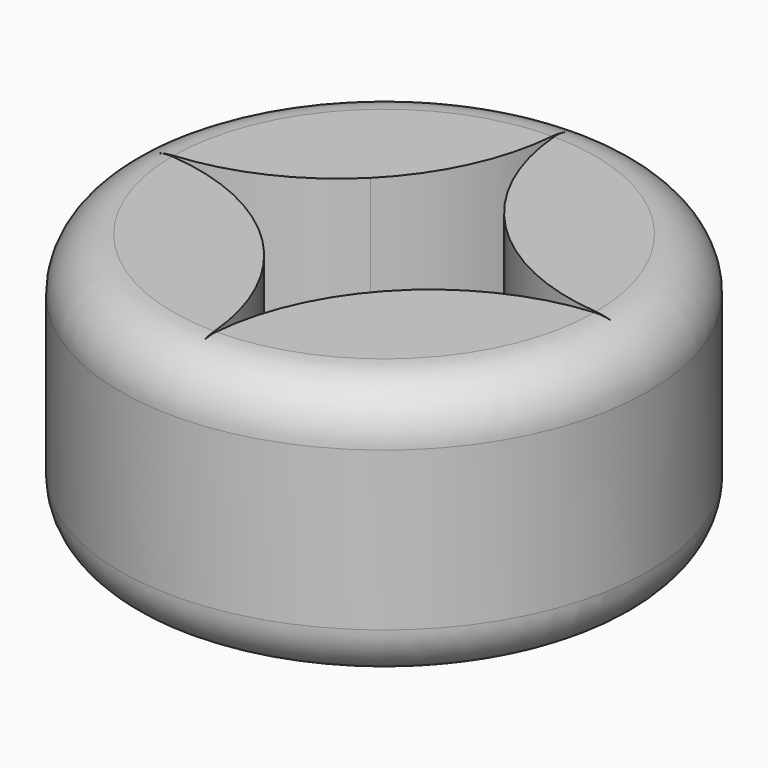
from build123d import *

# Parameters (mm, degrees)
F0_R     = 25.4
F1_DEPTH = 25.4


# Not quite as in the source:
# - a fillet or chamfer that OpenCascade refuses, or shapes differently, is made with other operations: its cross-section is extruded or revolved along the edge and cut away or added


with BuildPart() as f1:
    # F0 (on Top) → F1 (new body)
    with BuildSketch(Plane.XY):
        Circle(F0_R)
        with BuildLine():
            ThreePointArc((0, 22.225), (15.7154482119, 15.7154482119), (22.225, 0))
            ThreePointArc((22.225, 0), (15.7154482119, -15.7154482119), (0, -22.225))
            ThreePointArc((0, -22.225), (-15.7154482119, -15.7154482119), (-22.225, 0))
            ThreePointArc((-22.225, 0), (-15.7154482119, 15.7154482119), (0, 22.225))
        make_face(mode=Mode.SUBTRACT)
        with BuildLine():
            ThreePointArc((-6.5095517729, 6.5095518034), (-1.6917773858, 13.7198607256), (0, 22.225))
            ThreePointArc((0, 22.225), (-15.7154482119, 15.7154482119), (-22.225, 0))
            ThreePointArc((-22.225, 0), (-13.7198607057, 1.6917773941), (-6.5095517729, 6.5095518034))
        make_face()
        with BuildLine():
            ThreePointArc((6.509551813, 6.5095517633), (13.7198607319, 1.6917773832), (22.225, 0))
            ThreePointArc((22.225, 0), (15.7154482119, 15.7154482119), (0, 22.225))
            ThreePointArc((0, 22.225), (1.6917773967, 13.7198606994), (6.509551813, 6.5095517633))
        make_face()
        with BuildLine():
            ThreePointArc((-22.225, 0), (-15.7154482119, -15.7154482119), (0, -22.225))
            ThreePointArc((0, -22.225), (-1.6917773909, -13.7198607133), (-6.5095517917, -6.5095517845))
            ThreePointArc((-6.5095517917, -6.5095517845), (-13.719860718, -1.691777389), (-22.225, 0))
        make_face()
        with BuildLine():
            ThreePointArc((0, -22.225), (15.7154482119, -15.7154482119), (22.225, 0))
            ThreePointArc((22.225, 0), (13.7198607157, -1.6917773899), (6.5095517881, -6.5095517881))
            ThreePointArc((6.5095517881, -6.5095517881), (1.6917773899, -13.7198607157), (0, -22.225))
        make_face()
    extrude(amount=F1_DEPTH)

    # F2: fillet of radius 5.08 on 2 edges, made by hand

    # F2_s1 → F2_t2 (revolve, cut)
    with BuildSketch(Plane.XZ):
        with BuildLine():
            ThreePointArc((25.4, 20.32), (23.9121024484, 23.9121024484), (20.32, 25.4))
            Line((20.32, 25.4), (25.4, 25.4))
            Line((25.4, 25.4), (25.4, 20.32))
        make_face()
    revolve(axis=Axis((0, 0, 25.4), (0, 0, 1)), mode=Mode.SUBTRACT)

    # F2_s3 → F2_t4 (revolve, cut)
    with BuildSketch(Plane.XZ):
        with BuildLine():
            ThreePointArc((25.4, 5.08), (23.9121024484, 1.4878975516), (20.32, 0))
            Line((20.32, 0), (25.4, 0))
            Line((25.4, 0), (25.4, 5.08))
        make_face()
    revolve(axis=Axis((0, 0, 0), (0, 0, 1)), mode=Mode.SUBTRACT)


solid = f1.part
